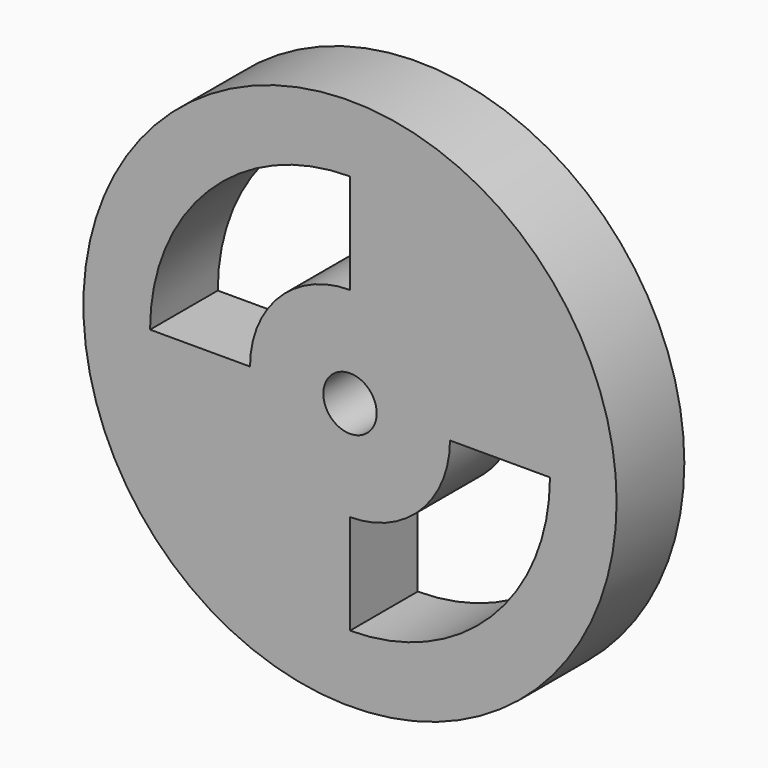
from build123d import *

# Parameters (mm, degrees)
F0_R     = 20
F0_R_2   = 2.0000994159
F1_DEPTH = 6.35


# Not quite as in the source:
# - a length typed as a fraction of an inch, garbled in the dataset ("3 / 203.2 mm" for 3/8 in), is restored


with BuildPart() as f1:
    # F0 (on Front) → F1 (new body)
    with BuildSketch(Plane.XZ):
        Circle(F0_R)
        with BuildLine():
            ThreePointArc((0, 15), (10.6066017178, 10.6066017178), (15, 0))
            ThreePointArc((15, 0), (10.6066017178, -10.6066017178), (0, -15))
            ThreePointArc((0, -15), (-10.6066017178, -10.6066017178), (-15, 0))
            ThreePointArc((-15, 0), (-10.6066017178, 10.6066017178), (0, 15))
        make_face(mode=Mode.SUBTRACT)
        with BuildLine():
            ThreePointArc((0, -7.5), (5.3033008589, -5.3033008589), (7.5, 0))
            ThreePointArc((7.5, 0), (5.3033008589, 5.3033008589), (0, 7.5))
            ThreePointArc((0, 7.5), (-5.3033008589, 5.3033008589), (-7.5, 0))
            ThreePointArc((-7.5, 0), (-5.3033008589, -5.3033008589), (0, -7.5))
        make_face()
        Circle(F0_R_2, mode=Mode.SUBTRACT)
        with BuildLine():
            ThreePointArc((-15, 0), (-10.6066017178, -10.6066017178), (0, -15))
            Line((0, -15), (0, -7.5))
            ThreePointArc((0, -7.5), (-5.3033008589, -5.3033008589), (-7.5, 0))
            Line((-7.5, 0), (-15, 0))
        make_face()
        with BuildLine():
            Line((7.5, 0), (15, 0))
            ThreePointArc((15, 0), (10.6066017178, 10.6066017178), (0, 15))
            Line((0, 15), (0, 7.5))
            ThreePointArc((0, 7.5), (5.3033008589, 5.3033008589), (7.5, 0))
        make_face()
    extrude(amount=F1_DEPTH)


solid = f1.part
